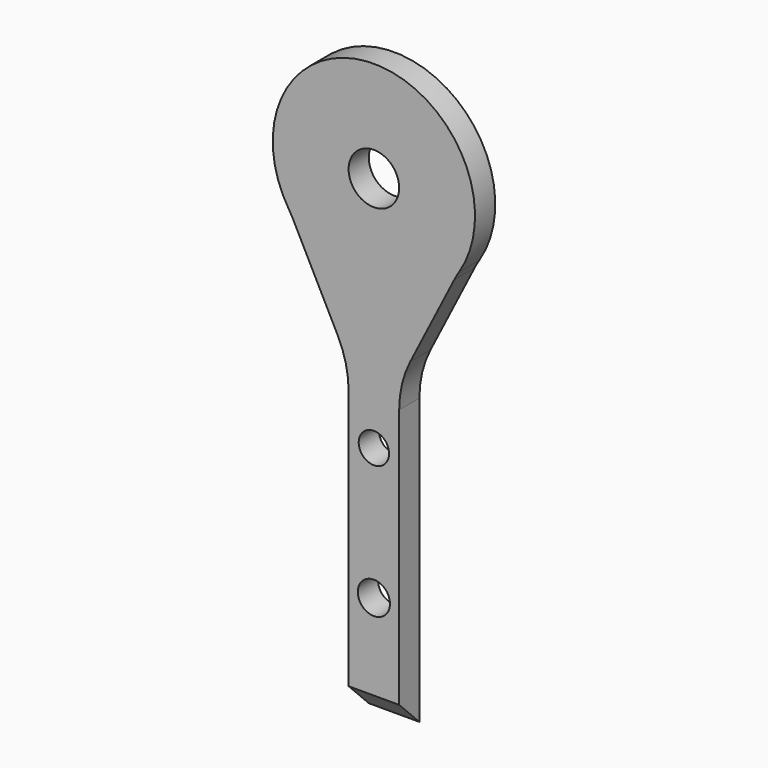
from build123d import *

# Parameters (mm, degrees)
F0_R        = 1.5
F0_R_2      = 1.5885930288
F0_R_3      = 2.5
F1_DEPTH    = 2.5
F2_T1_DEPTH = 30.7168298797
F3_R        = 10


# Not quite as in the source:
# - a fillet or chamfer that OpenCascade refuses, or shapes differently, is made with other operations: its cross-section is extruded or revolved along the edge and cut away or added


with BuildPart() as f1:
    # F0 (on Front) → F1 (new body)
    with BuildSketch(Plane.XZ):
        with BuildLine():
            Line((-0.0187197208, 13.0832688883), (5.6909857328, 24.2902945465))
            ThreePointArc((5.6909857328, 24.2902945465), (-2.5187197208, 40), (-10.7284251743, 24.2902945465))
            Line((-10.7284251743, 24.2902945465), (-5.0187197208, 13.0832688883))
            Line((-5.0187197208, 13.0832688883), (-5.0187197208, -20))
            Line((-5.0187197208, -20), (-0.0187197208, -20))
            Line((-0.0187197208, -20), (-0.0187197208, 13.0832688883))
        make_face()
        with Locations((-2.5187197208, 6.5416344441)):
            Circle(F0_R, mode=Mode.SUBTRACT)
        with Locations((-2.5187197208, -6.5)):
            Circle(F0_R_2, mode=Mode.SUBTRACT)
        with Locations((-2.5187197208, 30)):
            Circle(F0_R_3, mode=Mode.SUBTRACT)
    extrude(amount=F1_DEPTH)

    # F2: chamfer of 5 on 1 edges, made by hand

    # F2_s2 → F2_t1 (cut)
    with BuildSketch(Plane.YZ.offset(-17.8771346606)):
        Polygon((2.5, -20), (-2.5, -15), (-2.5, -20), align=None)
    extrude(amount=F2_T1_DEPTH, mode=Mode.SUBTRACT)

    # F3
    f3_edges = [f1.edges().sort_by_distance(p)[0] for p in [
        (-0.01872, -1.25, 13.083269),
        (-5.01872, -1.25, 13.083269),
        (5.690986, -1.25, 24.290295),
        (-10.728425, -1.25, 24.290295),
    ]]
    fillet(f3_edges, radius=F3_R)


solid = f1.part
